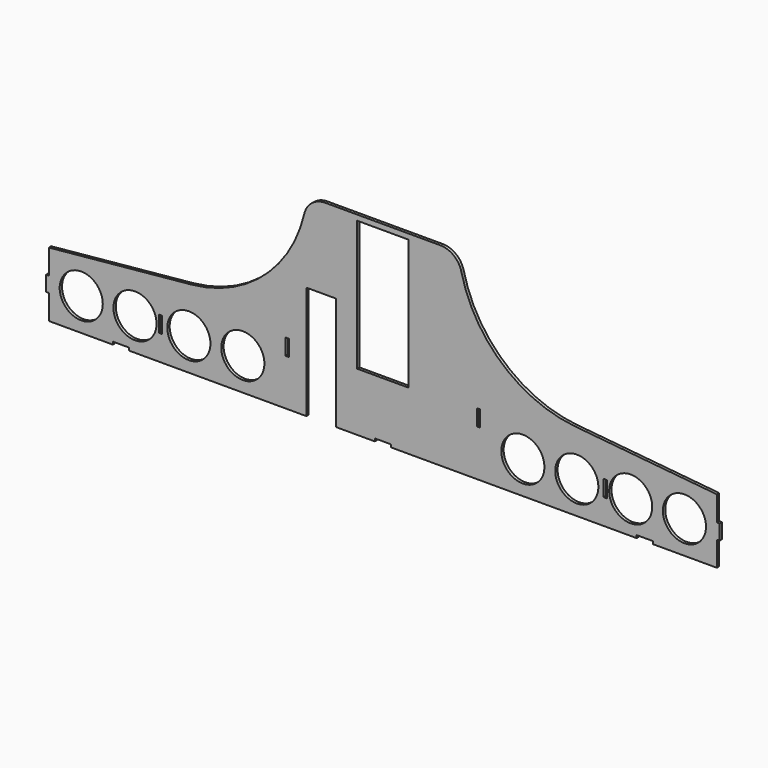
from build123d import *

# Parameters (mm, degrees)
F0_R     = 25.4
F0_W     = 3.81
F0_H     = 19.05
F0_W_2   = 60.325
F0_H_2   = 153.5942826
F1_DEPTH = 3.429


# Not quite as in the source:
# - ends of sketch curves that miss each other by under 0.0002 mm in the source are joined


with BuildPart() as f1:
    # F0 (on Front) → F1 (new body)
    with BuildSketch(Plane.XZ):
        with BuildLine():
            Line((68.2613062, -217.1147804), (68.2613062, -246.3247804))
            Line((68.2613062, -246.3247804), (143.8263062, -246.3247804))
            Line((143.8263062, -246.3247804), (143.8263062, -243.1497804))
            Line((143.8263062, -243.1497804), (162.8763062, -243.1497804))
            Line((162.8763062, -243.1497804), (162.8763062, -246.3247804))
            Line((162.8763062, -246.3247804), (371.7913062, -246.3247804))
            Line((371.7913062, -246.3247804), (371.7913062, -112.9747804))
            Line((371.7913062, -112.9747804), (406.7163062, -112.9747804))
            Line((406.7163062, -112.9747804), (406.7163062, -246.3247804))
            Line((406.7163062, -246.3247804), (452.4363062, -246.3247804))
            Line((452.4363062, -246.3247804), (452.4363062, -243.1497804))
            Line((452.4363062, -243.1497804), (471.4863062, -243.1497804))
            Line((471.4863062, -243.1497804), (471.4863062, -246.3247804))
            Line((471.4863062, -246.3247804), (761.0463062, -246.3247804))
            Line((761.0463062, -246.3247804), (761.0463062, -243.1497804))
            Line((761.0463062, -243.1497804), (780.0963062, -243.1497804))
            Line((780.0963062, -243.1497804), (780.0963062, -246.3247804))
            Line((780.0963062, -246.3247804), (855.6613062, -246.3247804))
            Line((855.6613062, -246.3247804), (855.6613062, -217.1147804))
            Line((855.6613062, -217.1147804), (858.8363062, -217.1147804))
            Line((858.8363062, -217.1147804), (858.8363062, -199.3347804))
            Line((858.8363062, -199.3347804), (855.6613062, -199.3347804))
            Line((855.6613062, -199.3347804), (855.6613062, -170.1247804))
            Line((855.6613062, -170.1247804), (688.2210772, -153.9405354))
            ThreePointArc((688.2210772, -153.9405354), (602.6698633523, -117.0648991424), (554.5656172379, -37.2851738969))
            ThreePointArc((554.5656172379, -37.2851738969), (545.6072798598, -23.2063701747), (529.846032, -17.7247804))
            Line((529.846032, -17.7247804), (394.0766058, -17.7247804))
            ThreePointArc((394.0766058, -17.7247804), (378.3153579402, -23.2063701747), (369.3569994588, -37.2851689116))
            ThreePointArc((369.3569994588, -37.2851689116), (321.2527512475, -117.0648972224), (235.7015357309, -153.9405408928))
            Line((235.7015357309, -153.9405408928), (68.2613062, -170.1247804))
            Line((68.2613062, -170.1247804), (68.2613062, -199.3347804))
            Line((68.2613062, -199.3347804), (65.0863062, -199.3347804))
            Line((65.0863062, -199.3347804), (65.0863062, -217.1147804))
            Line((65.0863062, -217.1147804), (68.2613062, -217.1147804))
        make_face()
        with Locations((106.5103026, -207.9172118)):
            Circle(F0_R, mode=Mode.SUBTRACT)
        with Locations((169.8620428, -207.9172118)):
            Circle(F0_R, mode=Mode.SUBTRACT)
        with Locations((199.9603062, -206.9547804)):
            Rectangle(F0_W, F0_H, mode=Mode.SUBTRACT)
        with Locations((233.3611284, -207.9172118)):
            Circle(F0_R, mode=Mode.SUBTRACT)
        with Locations((296.9567594, -207.9172118)):
            Circle(F0_R, mode=Mode.SUBTRACT)
        with Locations((349.1853062, -182.1897804)):
            Rectangle(F0_W, F0_H, mode=Mode.SUBTRACT)
        with Locations((626.9658784, -207.9172118)):
            Circle(F0_R, mode=Mode.SUBTRACT)
        with Locations((690.5615094, -207.9172118)):
            Circle(F0_R, mode=Mode.SUBTRACT)
        with Locations((723.9623062, -206.9547804)):
            Rectangle(F0_W, F0_H, mode=Mode.SUBTRACT)
        with Locations((754.0605696, -207.9172118)):
            Circle(F0_R, mode=Mode.SUBTRACT)
        with Locations((817.4123352, -207.9172118)):
            Circle(F0_R, mode=Mode.SUBTRACT)
        with Locations((574.7373062, -182.1897804)):
            Rectangle(F0_W, F0_H, mode=Mode.SUBTRACT)
        with Locations((461.9613062, -100.8605933)):
            Rectangle(F0_W_2, F0_H_2, mode=Mode.SUBTRACT)
    extrude(amount=F1_DEPTH)


solid = f1.part
